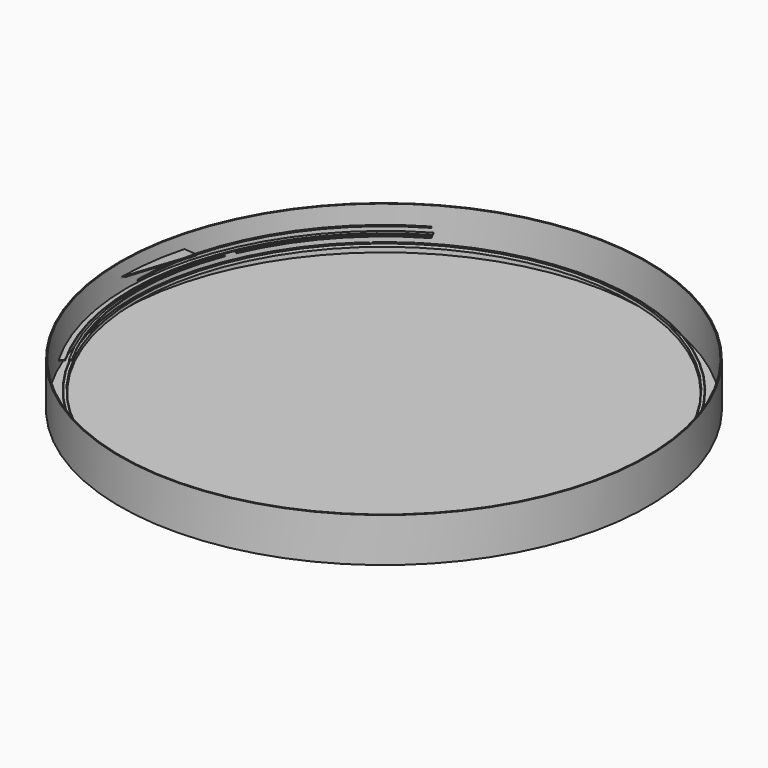
from build123d import *

# Parameters (mm, degrees)
F3_ANGLE_BACK = 30
F3_ANGLE      = 90
F5_ANGLE_BACK = 30
F5_ANGLE      = 90
F8_DEPTH      = 50.8
F9_ANGLE      = 60
F11_ANGLE     = 15
F12_DEPTH     = 871


# Not quite as in the source:
# - an extrude ends at something that could not be found from the text; its depth is read off the source's solid
# - a feature names something its author has since deleted; it is built from what else it names


with BuildPart() as f2:
    # F0 (on Front) → F2 (revolve)
    with BuildSketch(Plane.XZ):
        Polygon((-304.8, 22.2812721531), (-304.8, -3.1187278469), (-304.8, -28.5187278469), (0, -28.5187278469), (0, -27.2487278469), (-303.53, -27.2487278469), (-303.53, -4.0932331217), (-303.53, -2.7382071398), (-303.53, 5.5787864694), (-303.53, 6.8583239477), (-303.53, 22.2812721531), align=None)
    revolve(axis=Axis((0, 0, -10.9399985522), (0, 0, -1)))

    # F0 (on Front) → F11 (revolve)
    with BuildSketch(Plane.XZ):
        Polygon((-285.5563602362, 9.0652094139), (-303.53, 6.8583239477), (-303.53, 5.5787864694), (-285.5563602362, 7.7856719356), align=None)
    revolve(axis=Axis((0, 0, -10.9399985522), (0, 0, -1)), revolution_arc=F11_ANGLE)

    # F4 (on face) → F12 (cut, through all)
    with BuildSketch(Plane.XY.offset(-27.2487278469)):
        Polygon((-273.6640274525, 78.1679973006), (-303.53, 0), (-273.6640274525, -3.1685957219), align=None)
    extrude(amount=F12_DEPTH, mode=Mode.SUBTRACT)


with BuildPart() as f3:
    # F0 (on Front) → F3 (revolve)
    with BuildSketch(Plane.XZ, mode=Mode.PRIVATE) as f3_sk:
        Polygon((-290.83, -1.1788432163), (-296.672, -1.8961506211), (-296.5677402466, -2.7452781714), (-290.7257402466, -2.0279707666), align=None)
    revolve(f3_sk.sketch.rotate(Axis((0, 0, -10.9399985522), (0, 0, -1)), -F3_ANGLE_BACK), axis=Axis((0, 0, -10.9399985522), (0, 0, -1)), revolution_arc=F3_ANGLE)


with BuildPart() as f5:
    # F0 (on Front) → F5 (revolve)
    with BuildSketch(Plane.XZ, mode=Mode.PRIVATE) as f5_sk:
        Polygon((-284.6219958112, -1.2785251862), (-284.6219958112, -0.4165961479), (-287.3005058848, -0.7454758312), (-287.1962461314, -1.5946033814), align=None)
    revolve(f5_sk.sketch.rotate(Axis((0, 0, -10.9399985522), (0, 0, -1)), -F5_ANGLE_BACK), axis=Axis((0, 0, -10.9399985522), (0, 0, -1)), revolution_arc=F5_ANGLE)

    # F7 (on face) → F8 (cut)
    with BuildSketch(Plane.XY.offset(-27.2487278469)):
        Polygon((-263.6561095715, 114.8968338966), (-268.4032320976, 103.4207493067), (-263.9383698547, 102.0165755392), (-259.3476270111, 113.1146150174), align=None)
    extrude(amount=F8_DEPTH, mode=Mode.SUBTRACT)


with BuildPart() as f6:
    # F0 (on Front) → F6 (revolve)
    with BuildSketch(Plane.XZ):
        Polygon((-289.2928824048, -9.5292628156), (-289.7970958498, -9.5911724421), (-289.7661410366, -9.8432791646), (-289.2619275916, -9.7813695382), align=None)
    revolve(axis=Axis((0, 0, -10.9399985522), (0, 0, -1)))


with BuildPart() as f9:
    # F0 (on Front) → F9 (revolve)
    with BuildSketch(Plane.XZ):
        Polygon((-284.5823778866, 10.4643368874), (-284.8344846091, 10.4333820742), (-284.6797105429, 9.1728484616), (-284.4276038204, 9.2038032748), align=None)
    revolve(axis=Axis((0, 0, -10.9399985522), (0, 0, -1)), revolution_arc=F9_ANGLE)


with BuildPart() as f10:
    # F0 (on Front) → F10 (revolve)
    with BuildSketch(Plane.XZ):
        Polygon((-286.0154950121, -9.1268502437), (-286.2676017346, -9.1578050569), (-285.9215922653, -11.9758260426), (-285.8806665693, -12.3091390884), (-285.6285598468, -12.2781842752), align=None)
    revolve(axis=Axis((0, 0, -10.9399985522), (0, 0, -1)))


solid = Compound([f2.part, f3.part, f5.part, f6.part, f9.part, f10.part])
